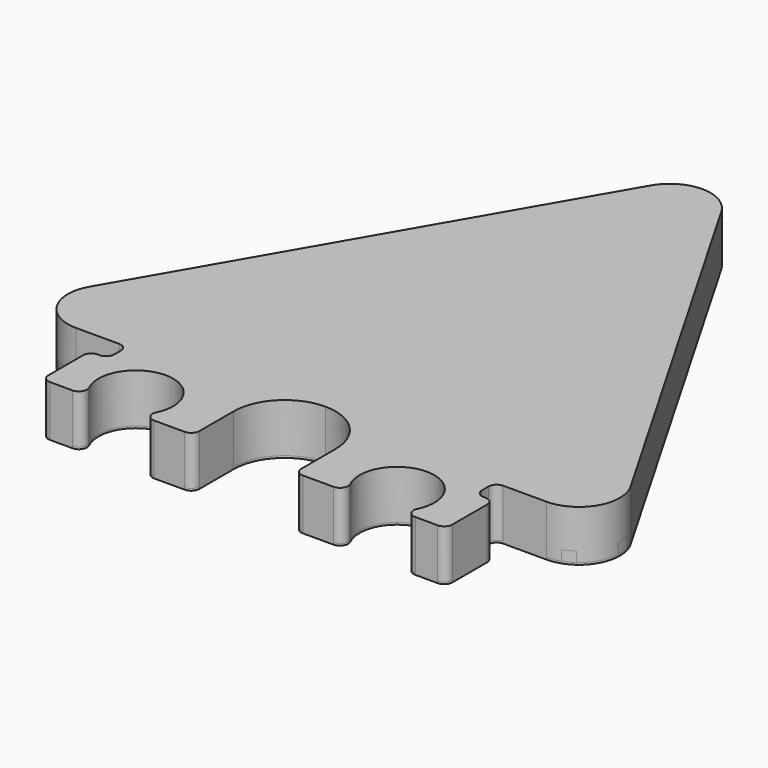
from build123d import *

# Parameters (mm, degrees)
F1_DEPTH = 4.8
F2_R     = 4
F4_DEPTH = 1
F5_DEPTH = 1
F6_R     = 0.8
F8_DEPTH = 0.2


# Not quite as in the source:
# - after a boolean that leaves OpenCascade's solid faulty, fix() repairs it


with BuildPart() as f1:
    # F0 (on Top) → F1 (new body)
    with BuildSketch(Plane.XY):
        with BuildLine():
            ThreePointArc((-5, 0), (-3.5355339059, 3.5355339059), (0, 5))
            ThreePointArc((0, 5), (3.5355339059, 3.5355339059), (5, 0))
            Line((5, 0), (5, -5))
            Line((5, -5), (10.4, -5))
            ThreePointArc((10.4, -5), (12.8088644564, 1.4307314955), (15.2177289128, -5))
            Line((15.2177289128, -5), (19.8177289128, -5))
            Line((19.8177289128, -5), (19.8177289128, 0.86))
            Line((19.8177289128, 0.86), (18.0377289128, 0.86))
            Line((18.0377289128, 0.86), (18.0377289128, 3.26))
            Line((18.0377289128, 3.26), (30, 3.26))
            Line((30, 3.26), (0, 55.2215242271))
            Line((0, 55.2215242271), (-30, 3.26))
            Line((-30, 3.26), (-18.0377289128, 3.26))
            Line((-18.0377289128, 3.26), (-18.0377289128, 0.86))
            Line((-18.0377289128, 0.86), (-19.8177289128, 0.86))
            Line((-19.8177289128, 0.86), (-19.8177289128, -5))
            Line((-19.8177289128, -5), (-15.2177289128, -5))
            ThreePointArc((-15.2177289128, -5), (-12.8088644564, 1.4307314955), (-10.4, -5))
            Line((-10.4, -5), (-5, -5))
            Line((-5, -5), (-5, 0))
        make_face()
    extrude(amount=F1_DEPTH)

    # F2
    f2_edges = [f1.edges().sort_by_distance(p)[0] for p in [
        (30, 3.26, 2.4),
        (0, 55.221524, 2.4),
        (-30, 3.26, 2.4),
    ]]
    fillet(f2_edges, radius=F2_R)

    # F3 (on face) → F4 (cut)
    with BuildSketch(Plane(origin=(0, 0, 0), x_dir=(1, 0, 0), z_dir=(0, 0, -1))):
        with BuildLine():
            Line((0, -9.7778161764), (0, -10.7778161764))
            Line((0, -10.7778161764), (13.737784962, -10.7778161764))
            Line((13.737784962, -10.7778161764), (25.4286516784, -4.0280911307))
            ThreePointArc((25.4286516784, -4.0280911307), (24.9241250755, -3.714738395), (24.3787619235, -3.4795447249))
            Line((24.3787619235, -3.4795447249), (13.4698357696, -9.7778161764))
            Line((13.4698357696, -9.7778161764), (0, -9.7778161764))
        make_face()
        with BuildLine():
            Line((-13.737784962, -10.7778161764), (0, -10.7778161764))
            Line((0, -10.7778161764), (0, -9.7778161764))
            Line((0, -9.7778161764), (-13.4698357696, -9.7778161764))
            Line((-13.4698357696, -9.7778161764), (-24.3787619235, -3.4795447249))
            ThreePointArc((-24.3787619235, -3.4795447249), (-24.9241250755, -3.714738395), (-25.4286516784, -4.0280911307))
            Line((-25.4286516784, -4.0280911307), (-13.737784962, -10.7778161764))
        make_face()
        with BuildLine():
            Line((1.7364629899, -37.1782497502), (1.7364629899, -50.8249526341))
            ThreePointArc((1.7364629899, -50.8249526341), (2.2626076246, -50.5201006984), (2.7364629899, -50.1390180668))
            Line((2.7364629899, -50.1390180668), (2.7364629899, -37.4461989427))
            Line((2.7364629899, -37.4461989427), (15.8779147563, -14.6845367981))
            Line((15.8779147563, -14.6845367981), (26.9338580546, -8.3013849587))
            ThreePointArc((26.9338580546, -8.3013849587), (27.0485392273, -7.6907196607), (27.0672656117, -7.0696615313))
            Line((27.0672656117, -7.0696615313), (15.1458639487, -13.9524859905))
            Line((15.1458639487, -13.9524859905), (1.7364629899, -37.1782497502))
        make_face()
        Polygon((8.4182686231, -15.72021842), (0, -15.72021842), (0, -16.8202612549), (6.5129385426, -16.8202612549), (0, -28.1010017173), (0, -30.301087387), align=None)
        Polygon((0, -16.8202612549), (0, -15.72021842), (-8.4182686231, -15.72021842), (0, -30.301087387), (0, -28.1010017173), (-6.5129385426, -16.8202612549), align=None)
        with BuildLine():
            Line((-15.1458639487, -13.9524859905), (-27.0672656117, -7.0696615313))
            ThreePointArc((-27.0672656117, -7.0696615313), (-27.0592311738, -7.5768073123), (-26.9870834272, -8.0788592001))
            ThreePointArc((-26.9870834272, -8.0788592001), (-26.962062144, -8.1905027231), (-26.9338580546, -8.3013849587))
            Line((-26.9338580546, -8.3013849587), (-15.8779147563, -14.6845367981))
            Line((-15.8779147563, -14.6845367981), (-2.7364629899, -37.4461989427))
            Line((-2.7364629899, -37.4461989427), (-2.7364629899, -50.1390180668))
            ThreePointArc((-2.7364629899, -50.1390180668), (-2.2626076246, -50.5201006984), (-1.7364629899, -50.8249526341))
            Line((-1.7364629899, -50.8249526341), (-1.7364629899, -37.1782497502))
            Line((-1.7364629899, -37.1782497502), (-15.1458639487, -13.9524859905))
        make_face()
    extrude(amount=-F4_DEPTH, mode=Mode.SUBTRACT)

    # F6
    f6_edges = [f1.edges().sort_by_distance(p)[0] for p in [
        (18.037729, 3.26, 2.4),
        (18.037729, 0.86, 2.4),
        (19.817729, 0.86, 2.4),
        (19.817729, -5, 2.4),
        (15.217729, -5, 2.4),
        (10.4, -5, 2.4),
        (5, -5, 2.4),
        (-5, -5, 2.4),
        (-10.4, -5, 2.4),
        (-15.217729, -5, 2.4),
        (-19.817729, -5, 2.4),
        (-19.817729, 0.86, 2.4),
        (-18.037729, 0.86, 2.4),
        (-18.037729, 3.26, 2.4),
    ]]
    fillet(f6_edges, radius=F6_R)

    # F7 (on face) → F8 (join)
    with BuildSketch(Plane(origin=(0, 0, 0), x_dir=(1, 0, 0), z_dir=(0, 0, -1))):
        with BuildLine():
            Line((3.4641016151, -49.2215242271), (26.5358983849, -9.26))
            ThreePointArc((26.5358983849, -9.26), (26.7661033905, -8.793655304), (26.9338580546, -8.3013849587))
            ThreePointArc((26.9338580546, -8.3013849587), (27.0485392273, -7.6907196607), (27.0672656117, -7.0696615313))
            ThreePointArc((27.0672656117, -7.0696615313), (26.5932725802, -5.3628420951), (25.4286516784, -4.0280911307))
            ThreePointArc((25.4286516784, -4.0280911307), (24.9241250755, -3.714738395), (24.3787619235, -3.4795447249))
            Line((24.3787619235, -3.4795447249), (13.4698357696, -9.7778161764))
            Line((13.4698357696, -9.7778161764), (-13.4698357696, -9.7778161764))
            Line((-13.4698357696, -9.7778161764), (-24.3787619235, -3.4795447249))
            ThreePointArc((-24.3787619235, -3.4795447249), (-24.9241250755, -3.714738395), (-25.4286516784, -4.0280911307))
            ThreePointArc((-25.4286516784, -4.0280911307), (-26.5932725802, -5.3628420951), (-27.0672656117, -7.0696615313))
            ThreePointArc((-27.0672656117, -7.0696615313), (-27.0485392273, -7.6907196607), (-26.9338580546, -8.3013849587))
            ThreePointArc((-26.9338580546, -8.3013849587), (-26.7661033905, -8.793655304), (-26.5358983849, -9.26))
            Line((-26.5358983849, -9.26), (-3.4641016151, -49.2215242271))
            ThreePointArc((-3.4641016151, -49.2215242271), (-3.1340387828, -49.7070424644), (-2.7364629899, -50.1390180668))
            ThreePointArc((-2.7364629899, -50.1390180668), (-2.2626076246, -50.5201006984), (-1.7364629899, -50.8249526341))
            ThreePointArc((-1.7364629899, -50.8249526341), (0, -51.2215242271), (1.7364629899, -50.8249526341))
            ThreePointArc((1.7364629899, -50.8249526341), (2.2626076246, -50.5201006984), (2.7364629899, -50.1390180668))
            ThreePointArc((2.7364629899, -50.1390180668), (3.1340387828, -49.7070424644), (3.4641016151, -49.2215242271))
        make_face()
        with BuildLine():
            Line((13.4698357696, -9.7778161764), (24.3787619235, -3.4795447249))
            ThreePointArc((24.3787619235, -3.4795447249), (23.7344350193, -3.3152680002), (23.0717967697, -3.26))
            Line((23.0717967697, -3.26), (18.8377289128, -3.26))
            ThreePointArc((18.8377289128, -3.26), (18.2720434879, -3.0256854249), (18.0377289128, -2.46))
            Line((18.0377289128, -2.46), (18.0377289128, -1.66))
            ThreePointArc((18.0377289128, -1.66), (18.2720434879, -1.0943145751), (18.8377289128, -0.86))
            Line((18.8377289128, -0.86), (19.0177289128, -0.86))
            ThreePointArc((19.0177289128, -0.86), (19.5834143378, -0.6256854249), (19.8177289128, -0.06))
            Line((19.8177289128, -0.06), (19.8177289128, 4.2))
            ThreePointArc((19.8177289128, 4.2), (19.5834143378, 4.7656854249), (19.0177289128, 5))
            Line((19.0177289128, 5), (16.8203228399, 5))
            ThreePointArc((16.8203228399, 5), (16.1415568612, 4.623410848), (16.1018306433, 3.8481918655))
            ThreePointArc((16.1018306433, 3.8481918655), (12.8088644564, -1.4307314955), (9.5158982695, 3.8481918655))
            ThreePointArc((9.5158982695, 3.8481918655), (9.4761720516, 4.623410848), (8.797406073, 5))
            Line((8.797406073, 5), (5.8, 5))
            ThreePointArc((5.8, 5), (5.2343145751, 4.7656854249), (5, 4.2))
            Line((5, 4.2), (5, 0))
            ThreePointArc((5, 0), (0, -5), (-5, 0))
            Line((-5, 0), (-5, 4.2))
            ThreePointArc((-5, 4.2), (-5.2343145751, 4.7656854249), (-5.8, 5))
            Line((-5.8, 5), (-8.797406073, 5))
            ThreePointArc((-8.797406073, 5), (-9.4761720516, 4.623410848), (-9.5158982695, 3.8481918655))
            ThreePointArc((-9.5158982695, 3.8481918655), (-12.8088644564, -1.4307314955), (-16.1018306433, 3.8481918655))
            ThreePointArc((-16.1018306433, 3.8481918655), (-16.1415568612, 4.623410848), (-16.8203228399, 5))
            Line((-16.8203228399, 5), (-19.0177289128, 5))
            ThreePointArc((-19.0177289128, 5), (-19.5834143378, 4.7656854249), (-19.8177289128, 4.2))
            Line((-19.8177289128, 4.2), (-19.8177289128, -0.06))
            ThreePointArc((-19.8177289128, -0.06), (-19.5834143378, -0.6256854249), (-19.0177289128, -0.86))
            Line((-19.0177289128, -0.86), (-18.8377289128, -0.86))
            ThreePointArc((-18.8377289128, -0.86), (-18.2720434879, -1.0943145751), (-18.0377289128, -1.66))
            Line((-18.0377289128, -1.66), (-18.0377289128, -2.46))
            ThreePointArc((-18.0377289128, -2.46), (-18.2720434879, -3.0256854249), (-18.8377289128, -3.26))
            Line((-18.8377289128, -3.26), (-23.0717967697, -3.26))
            ThreePointArc((-23.0717967697, -3.26), (-23.7344350193, -3.3152680002), (-24.3787619235, -3.4795447249))
            Line((-24.3787619235, -3.4795447249), (-13.4698357696, -9.7778161764))
            Line((-13.4698357696, -9.7778161764), (13.4698357696, -9.7778161764))
        make_face()
    extrude(amount=F8_DEPTH)

    add(f1.part.fix(), mode=Mode.REPLACE)


with BuildPart() as f5:
    # F3 (on face) → F5 (new body)
    with BuildSketch(Plane(origin=(0, 0, 0), x_dir=(1, 0, 0), z_dir=(0, 0, -1))):
        with BuildLine():
            Line((0, -9.7778161764), (0, -10.7778161764))
            Line((0, -10.7778161764), (13.737784962, -10.7778161764))
            Line((13.737784962, -10.7778161764), (25.4286516784, -4.0280911307))
            ThreePointArc((25.4286516784, -4.0280911307), (24.9241250755, -3.714738395), (24.3787619235, -3.4795447249))
            Line((24.3787619235, -3.4795447249), (13.4698357696, -9.7778161764))
            Line((13.4698357696, -9.7778161764), (0, -9.7778161764))
        make_face()
        with BuildLine():
            Line((-13.737784962, -10.7778161764), (0, -10.7778161764))
            Line((0, -10.7778161764), (0, -9.7778161764))
            Line((0, -9.7778161764), (-13.4698357696, -9.7778161764))
            Line((-13.4698357696, -9.7778161764), (-24.3787619235, -3.4795447249))
            ThreePointArc((-24.3787619235, -3.4795447249), (-24.9241250755, -3.714738395), (-25.4286516784, -4.0280911307))
            Line((-25.4286516784, -4.0280911307), (-13.737784962, -10.7778161764))
        make_face()
    extrude(amount=-F5_DEPTH)


with BuildPart() as f5b:
    # F3 (on face) → F5, piece 2 (new body)
    with BuildSketch(Plane(origin=(0, 0, 0), x_dir=(1, 0, 0), z_dir=(0, 0, -1))):
        with BuildLine():
            Line((1.7364629899, -37.1782497502), (1.7364629899, -50.8249526341))
            ThreePointArc((1.7364629899, -50.8249526341), (2.2626076246, -50.5201006984), (2.7364629899, -50.1390180668))
            Line((2.7364629899, -50.1390180668), (2.7364629899, -37.4461989427))
            Line((2.7364629899, -37.4461989427), (15.8779147563, -14.6845367981))
            Line((15.8779147563, -14.6845367981), (26.9338580546, -8.3013849587))
            ThreePointArc((26.9338580546, -8.3013849587), (27.0485392273, -7.6907196607), (27.0672656117, -7.0696615313))
            Line((27.0672656117, -7.0696615313), (15.1458639487, -13.9524859905))
            Line((15.1458639487, -13.9524859905), (1.7364629899, -37.1782497502))
        make_face()
    extrude(amount=-F5_DEPTH)


with BuildPart() as f5c:
    # F3 (on face) → F5, piece 3 (new body)
    with BuildSketch(Plane(origin=(0, 0, 0), x_dir=(1, 0, 0), z_dir=(0, 0, -1))):
        Polygon((8.4182686231, -15.72021842), (0, -15.72021842), (0, -16.8202612549), (6.5129385426, -16.8202612549), (0, -28.1010017173), (0, -30.301087387), align=None)
        Polygon((0, -16.8202612549), (0, -15.72021842), (-8.4182686231, -15.72021842), (0, -30.301087387), (0, -28.1010017173), (-6.5129385426, -16.8202612549), align=None)
    extrude(amount=-F5_DEPTH)


with BuildPart() as f5d:
    # F3 (on face) → F5, piece 4 (new body)
    with BuildSketch(Plane(origin=(0, 0, 0), x_dir=(1, 0, 0), z_dir=(0, 0, -1))):
        with BuildLine():
            Line((-15.1458639487, -13.9524859905), (-27.0672656117, -7.0696615313))
            ThreePointArc((-27.0672656117, -7.0696615313), (-27.0592311738, -7.5768073123), (-26.9870834272, -8.0788592001))
            ThreePointArc((-26.9870834272, -8.0788592001), (-26.962062144, -8.1905027231), (-26.9338580546, -8.3013849587))
            Line((-26.9338580546, -8.3013849587), (-15.8779147563, -14.6845367981))
            Line((-15.8779147563, -14.6845367981), (-2.7364629899, -37.4461989427))
            Line((-2.7364629899, -37.4461989427), (-2.7364629899, -50.1390180668))
            ThreePointArc((-2.7364629899, -50.1390180668), (-2.2626076246, -50.5201006984), (-1.7364629899, -50.8249526341))
            Line((-1.7364629899, -50.8249526341), (-1.7364629899, -37.1782497502))
            Line((-1.7364629899, -37.1782497502), (-15.1458639487, -13.9524859905))
        make_face()
    extrude(amount=-F5_DEPTH)


solid = Compound([f1.part, f5.part, f5b.part, f5c.part, f5d.part])
